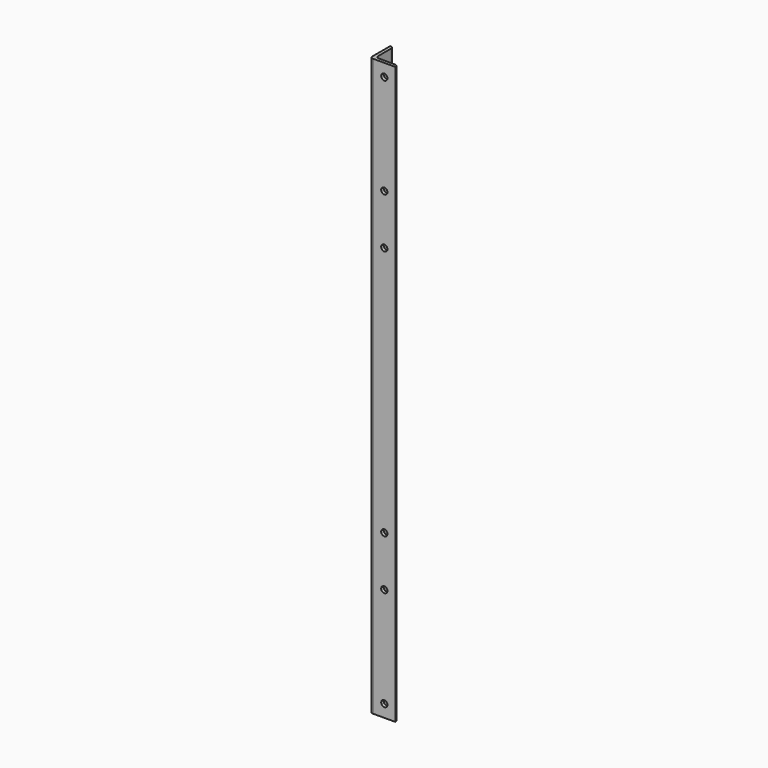
from build123d import *

# Parameters (mm, degrees)
F1_DEPTH    = 584.2
F2_R        = 3.175
F3_DEPTH    = 3.175
F4_R        = 3.175
F5_DEPTH    = 25.4
F6_T1_DEPTH = 600.075
F7_T1_DEPTH = 584.2
F7_T3_DEPTH = 600.075
F8_R        = 3.175
F9_DEPTH    = 3.175


# Not quite as in the source:
# - a fillet or chamfer that OpenCascade refuses, or shapes differently, is made with other operations: its cross-section is extruded or revolved along the edge and cut away or added


with BuildPart() as f1:
    # F0 (on Top) → F1 (new body)
    with BuildSketch(Plane.XY):
        Polygon((-18.6830897415, 6.6160263166), (-21.8580897415, 6.6160263166), (-21.8580897415, -18.7839736834), (3.5419102585, -18.7839736834), (3.5419102585, -15.6089736834), (-18.6830897415, -15.6089736834), align=None)
    extrude(amount=F1_DEPTH)

    # F2 (on face) → F3 (cut)
    with BuildSketch(Plane.YZ.offset(-18.6830897415)):
        with Locations((-4.4964736834, 571.5)):
            Circle(F2_R)
        with Locations((-4.4964736834, 12.7)):
            Circle(F2_R)
    extrude(amount=-F3_DEPTH, mode=Mode.SUBTRACT)

    # F4 (on face) → F5 (cut)
    with BuildSketch(Plane(origin=(0, -15.6089736834, 0), x_dir=(-1, 0, 0), z_dir=(0, 1, 0))):
        with Locations((7.5705897415, 12.7)):
            Circle(F4_R)
        with Locations((7.5705897415, 571.5)):
            Circle(F4_R)
    extrude(amount=-F5_DEPTH, mode=Mode.SUBTRACT)

    # F6: fillet of radius 3.175 on 2 edges, made by hand

    # F6_s2 → F6_t1 (cut)
    with BuildSketch(Plane.XY.offset(-7.9375)):
        with BuildLine():
            add(Edge.make_bspline(
                [(0.3669102585, -15.6089736834), (3.5419102585, -15.6089736834), (3.5419102585, -18.7839736834)],
                knots=[0, 0, 0, 1, 1, 1], degree=2, weights=[1, 1, 1]))
            Line((3.5419102585, -18.7839736834), (3.5419102585, -15.6089736834))
            Line((3.5419102585, -15.6089736834), (0.3669102585, -15.6089736834))
        make_face()
        with BuildLine():
            add(Edge.make_bspline(
                [(-18.6830897415, 3.4410263166), (-18.6830897415, 6.6160263166), (-21.8580897415, 6.6160263166)],
                knots=[0, 0, 0, 1, 1, 1], degree=2, weights=[1, 1, 1]))
            Line((-21.8580897415, 6.6160263166), (-18.6830897415, 6.6160263166))
            Line((-18.6830897415, 6.6160263166), (-18.6830897415, 3.4410263166))
        make_face()
    extrude(amount=F6_T1_DEPTH, mode=Mode.SUBTRACT)

    # F7: fillet of radius 3.175 on 2 edges, made by hand

    # F7_s2 → F7_t1 (join)
    with BuildSketch(Plane.XY):
        with BuildLine():
            add(Edge.make_bspline(
                [(-18.6830897415, -12.4339736834), (-18.6830897415, -15.6089736834), (-15.5080897415, -15.6089736834)],
                knots=[0, 0, 0, 1, 1, 1], degree=2, weights=[1, 1, 1]))
            Line((-15.5080897415, -15.6089736834), (-18.6830897415, -15.6089736834))
            Line((-18.6830897415, -15.6089736834), (-18.6830897415, -12.4339736834))
        make_face()
    extrude(amount=F7_T1_DEPTH)

    # F7_s4 → F7_t3 (cut)
    with BuildSketch(Plane.XY.offset(-7.9375)):
        with BuildLine():
            add(Edge.make_bspline(
                [(-18.6830897415, -18.7839736834), (-21.8580897415, -18.7839736834), (-21.8580897415, -15.6089736834)],
                knots=[0, 0, 0, 1, 1, 1], degree=2, weights=[1, 1, 1]))
            Line((-21.8580897415, -15.6089736834), (-21.8580897415, -18.7839736834))
            Line((-21.8580897415, -18.7839736834), (-18.6830897415, -18.7839736834))
        make_face()
    extrude(amount=F7_T3_DEPTH, mode=Mode.SUBTRACT)

    # F8 (on face) → F9 (cut)
    with BuildSketch(Plane(origin=(0, -15.6089736834, 0), x_dir=(-1, 0, 0), z_dir=(0, 1, 0))):
        with Locations((7.5705897415, 165.1)):
            Circle(F8_R)
        with Locations((7.5705897415, 114.3)):
            Circle(F8_R)
        with Locations((7.5705897415, 469.9)):
            Circle(F8_R)
        with Locations((7.5705897415, 419.1)):
            Circle(F8_R)
    extrude(amount=-F9_DEPTH, mode=Mode.SUBTRACT)


solid = f1.part
